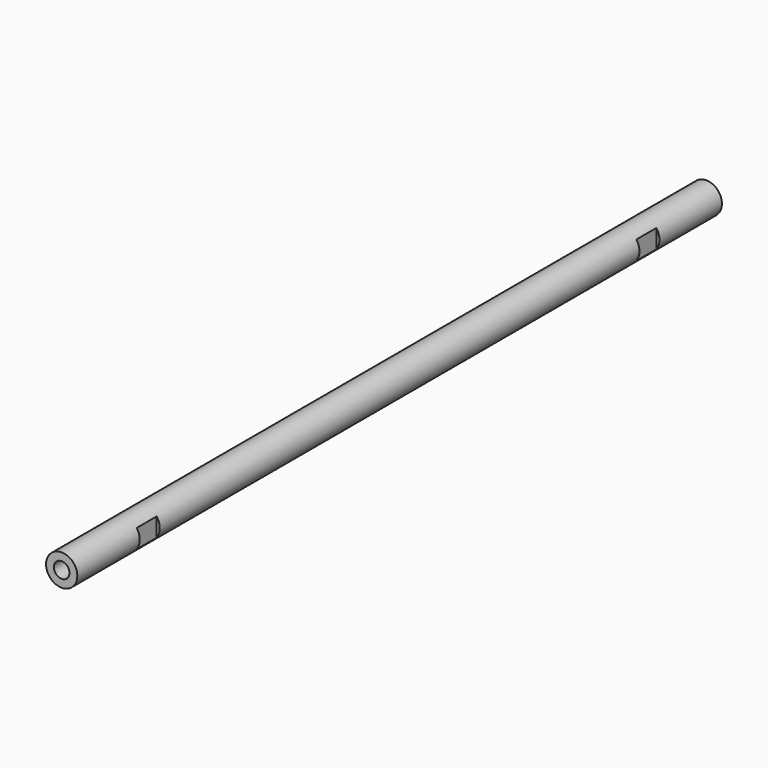
from build123d import *

# Parameters (mm, degrees)
F0_R     = 5
F1_DEPTH = 129
F3_D     = 5
F3_DEPTH = 35
F3_TIP   = 1.5021515476
F5_D     = 5
F5_DEPTH = 35
F5_TIP   = 1.5021515476
F8_DEPTH = 8


# Not quite as in the source:
# - a pattern or mirror of a feature is missing from the dataset's text; its kind, count and spacing are read off the source's solid


with BuildPart() as f1:
    # F0 (on Front) → F1 (new body, symmetric)
    with BuildSketch(Plane.XZ):
        Circle(F0_R)
    extrude(amount=F1_DEPTH, both=True)

    # F3
    with Locations(Plane.XZ.offset(129)):
        with Locations((0, 0)):
            Hole(F3_D / 2, depth=F3_DEPTH)
            with Locations((0, 0, -(F3_DEPTH + F3_TIP / 2))):  # 118° drill point
                Cone(0, F3_D / 2, F3_TIP, mode=Mode.SUBTRACT)

    # F5
    with Locations(Plane(origin=(0, 129, 0), x_dir=(-1, 0, 0), z_dir=(0, 1, 0))):
        with Locations((0, 0)):
            Hole(F5_D / 2, depth=F5_DEPTH)
            with Locations((0, 0, -(F5_DEPTH + F5_TIP / 2))):  # 118° drill point
                Cone(0, F5_D / 2, F5_TIP, mode=Mode.SUBTRACT)

    # F7 (on offset) → F8 (cut)
    with BuildSketch(Plane.XZ.offset(104)):
        with BuildLine():
            Line((-4, -3), (-4, 3))
            ThreePointArc((-4, 3), (-5, 0), (-4, -3))
        make_face()
        with BuildLine():
            ThreePointArc((5, 0), (4.7434164903, 1.5811388301), (4, 3))
            Line((4, 3), (4, -3))
            ThreePointArc((4, -3), (4.7434164903, -1.5811388301), (5, 0))
        make_face()
    f8 = extrude(amount=-F8_DEPTH, mode=Mode.SUBTRACT)

    # F8_copies: F8 across plane
    add(f8.mirror(Plane.ZX), mode=Mode.SUBTRACT)


solid = f1.part
